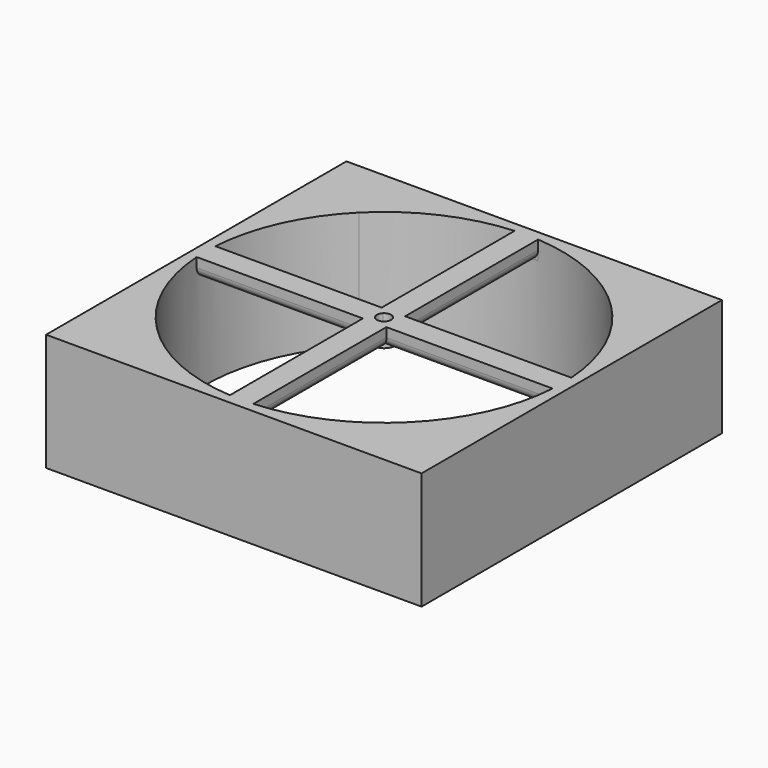
from build123d import *

# Parameters (mm, degrees)
F0_W          = 80
F0_H          = 80
F1_DEPTH      = 25
F3_DEPTH      = 25
F4_W          = 37.5
F4_H          = 5
F4_W_2        = 5
F4_H_2        = 37.5
F5_DEPTH      = 4
F6_T4_DEPTH   = 40.4176739793
F6_S5_R       = 38
F6_T6_DEPTH   = 22
F6_T10_DEPTH  = 40.4176739793
F6_S11_R      = 38
F6_T12_DEPTH  = 22
F6_T16_DEPTH  = 40.4176739793
F6_S17_R      = 38
F6_T18_DEPTH  = 22
F6_T22_DEPTH  = 40.4176739793
F6_S23_R      = 38
F6_T24_DEPTH  = 22
F6_T28_DEPTH  = 40.4176739793
F6_S29_R      = 38
F6_T30_DEPTH  = 22
F6_T34_DEPTH  = 40.4176739793
F6_S35_R      = 38
F6_T36_DEPTH  = 22
F6_T40_DEPTH  = 40.4176739793
F6_S41_R      = 38
F6_T42_DEPTH  = 22
F6_T46_DEPTH  = 40.4176739793
F6_S47_R      = 38
F6_T48_DEPTH  = 22
F6_T53_DEPTH  = 45.4176739793
F6_S54_R      = 1.5
F6_T55_DEPTH  = 24
F6_T59_DEPTH  = 45.4176739793
F6_S60_R      = 1.5
F6_T61_DEPTH  = 24
F6_T68_DEPTH  = 45.4176739793
F6_S69_R      = 1.5
F6_T70_DEPTH  = 24
F6_T74_DEPTH  = 45.4176739793
F6_S75_R      = 1.5
F6_T76_DEPTH  = 24
F6_T83_DEPTH  = 45.4176739793
F6_S85_R      = 1.5
F6_T86_DEPTH  = 24
F6_T89_DEPTH  = 45.4176739793
F6_S91_R      = 1.5
F6_T92_DEPTH  = 24
F6_T98_DEPTH  = 45.4176739793
F6_S99_R      = 1.5
F6_T100_DEPTH = 24
F6_T104_DEPTH = 45.4176739793
F6_S105_R     = 1.5
F6_T106_DEPTH = 24
F7_R          = 2.4952367962
F8_DEPTH      = 0.5


# Not quite as in the source:
# - a fillet or chamfer that OpenCascade refuses, or shapes differently, is made with other operations: its cross-section is extruded or revolved along the edge and cut away or added


with BuildPart() as f1:
    # F0 (on Top) → F1 (new body)
    with BuildSketch(Plane.XY):
        with Locations((-5.8039426804, 2.9257544003)):
            Rectangle(F0_W, F0_H)
    extrude(amount=F1_DEPTH)

    # F2 (on face) → F3 (cut)
    with BuildSketch(Plane.XY.offset(25)):
        with BuildLine():
            ThreePointArc((21.0661150047, 29.7958120854), (-5.8039426804, 40.9257544003), (-32.6740003654, 29.7958120854))
            Line((-32.6740003654, 29.7958120854), (-5.8039426804, 2.9257544003))
            Line((-5.8039426804, 2.9257544003), (21.0661150047, 29.7958120854))
        make_face()
        with BuildLine():
            Line((-5.8039426804, 2.9257544003), (-32.6740003654, 29.7958120854))
            ThreePointArc((-32.6740003654, 29.7958120854), (-43.8039426804, 2.9257544003), (-32.6740003654, -23.9443032848))
            Line((-32.6740003654, -23.9443032848), (-5.8039426804, 2.9257544003))
        make_face()
        with BuildLine():
            Line((21.0661150047, 29.7958120854), (-5.8039426804, 2.9257544003))
            Line((-5.8039426804, 2.9257544003), (21.0661150047, -23.9443032848))
            ThreePointArc((21.0661150047, -23.9443032848), (29.3034795551, -11.6162160296), (32.1960573196, 2.9257544003))
            ThreePointArc((32.1960573196, 2.9257544003), (29.3034795551, 17.4677248302), (21.0661150047, 29.7958120854))
        make_face()
        with BuildLine():
            Line((21.0661150047, -23.9443032848), (-5.8039426804, 2.9257544003))
            Line((-5.8039426804, 2.9257544003), (-32.6740003654, -23.9443032848))
            ThreePointArc((-32.6740003654, -23.9443032848), (-5.8039426804, -35.0742455997), (21.0661150047, -23.9443032848))
        make_face()
    extrude(amount=-F3_DEPTH, mode=Mode.SUBTRACT)

    # F4 (on face) → F5 (join)
    with BuildSketch(Plane.XY.offset(25)):
        Polygon((-8.3039426804, -37.0742455997), (-5.8039426804, -37.0742455997), (-3.3039426804, -37.0742455997), (-3.3039426804, 0.4257544003), (-8.3039426804, 0.4257544003), align=None)
        with Locations((-27.0539426804, 2.9257544003)):
            Rectangle(F4_W, F4_H)
        with BuildLine():
            Line((-6.8646028521, 1.8650942285), (-8.3039426804, 0.4257544003))
            Line((-8.3039426804, 0.4257544003), (-3.3039426804, 0.4257544003))
            Line((-3.3039426804, 0.4257544003), (-4.7432825086, 1.8650942285))
            ThreePointArc((-4.7432825086, 1.8650942285), (-5.8039426804, 1.4257544003), (-6.8646028521, 1.8650942285))
        make_face()
        with BuildLine():
            Line((-8.3039426804, 5.4257544003), (-8.3039426804, 0.4257544003))
            Line((-8.3039426804, 0.4257544003), (-6.8646028521, 1.8650942285))
            ThreePointArc((-6.8646028521, 1.8650942285), (-7.3039426804, 2.9257544003), (-6.8646028521, 3.9864145721))
            Line((-6.8646028521, 3.9864145721), (-8.3039426804, 5.4257544003))
        make_face()
        with BuildLine():
            Line((-4.7432825086, 1.8650942285), (-3.3039426804, 0.4257544003))
            Line((-3.3039426804, 0.4257544003), (-3.3039426804, 5.4257544003))
            Line((-3.3039426804, 5.4257544003), (-4.7432825086, 3.9864145721))
            ThreePointArc((-4.7432825086, 3.9864145721), (-4.4181233816, 3.4997795488), (-4.3039426804, 2.9257544003))
            ThreePointArc((-4.3039426804, 2.9257544003), (-4.4181233816, 2.3517292517), (-4.7432825086, 1.8650942285))
        make_face()
        with Locations((15.4460573196, 2.9257544003)):
            Rectangle(F4_W, F4_H)
        with Locations((-5.8039426804, 24.1757544003)):
            Rectangle(F4_W_2, F4_H_2)
        with BuildLine():
            Line((-3.3039426804, 5.4257544003), (-8.3039426804, 5.4257544003))
            Line((-8.3039426804, 5.4257544003), (-6.8646028521, 3.9864145721))
            ThreePointArc((-6.8646028521, 3.9864145721), (-5.8039426804, 4.4257544003), (-4.7432825086, 3.9864145721))
            Line((-4.7432825086, 3.9864145721), (-3.3039426804, 5.4257544003))
        make_face()
    extrude(amount=-F5_DEPTH)

    # F6: fillet of radius 2 on 8 edges, made by hand


with BuildPart() as f6_tool2:
    # F6_s3 → F6_t4 (new body)
    with BuildSketch(Plane.XZ.offset(-5.4257544003)):
        with BuildLine():
            ThreePointArc((-5.3039426804, 21), (-3.889729118, 21.5857864376), (-3.3039426804, 23))
            Line((-3.3039426804, 23), (-3.3039426804, 21))
            Line((-3.3039426804, 21), (-5.3039426804, 21))
        make_face()
    extrude(amount=-F6_T4_DEPTH)

    # F6_s5 → F6_t6 (intersect, symmetric)
    with BuildSketch(Plane.XY.offset(22)):
        with Locations((-5.8039426804, 2.9257544003)):
            Circle(F6_S5_R)
    extrude(amount=F6_T6_DEPTH, both=True, mode=Mode.INTERSECT)


with BuildPart() as f1_1:
    add(f1.part)

    # F6_t1: cut F6_tool2
    add(f6_tool2.part, mode=Mode.SUBTRACT)


with BuildPart() as f6_tool8:
    # F6_s9 → F6_t10 (new body)
    with BuildSketch(Plane.XZ.offset(-0.4257544003)):
        with BuildLine():
            ThreePointArc((-6.3039426804, 21), (-7.7181562427, 21.5857864376), (-8.3039426804, 23))
            Line((-8.3039426804, 23), (-8.3039426804, 21))
            Line((-8.3039426804, 21), (-6.3039426804, 21))
        make_face()
    extrude(amount=F6_T10_DEPTH)

    # F6_s11 → F6_t12 (intersect, symmetric)
    with BuildSketch(Plane.XY.offset(22)):
        with Locations((-5.8039426804, 2.9257544003)):
            Circle(F6_S11_R)
    extrude(amount=F6_T12_DEPTH, both=True, mode=Mode.INTERSECT)


with BuildPart() as f1_2:
    add(f1_1.part)

    # F6_t7: cut F6_tool8
    add(f6_tool8.part, mode=Mode.SUBTRACT)


with BuildPart() as f6_tool14:
    # F6_s15 → F6_t16 (new body)
    with BuildSketch(Plane.YZ.offset(-48.7216166597)):
        with BuildLine():
            ThreePointArc((2.4257544003, 21), (1.0115408379, 21.5857864376), (0.4257544003, 23))
            Line((0.4257544003, 23), (0.4257544003, 21))
            Line((0.4257544003, 21), (2.4257544003, 21))
        make_face()
    extrude(amount=F6_T16_DEPTH)

    # F6_s17 → F6_t18 (intersect, symmetric)
    with BuildSketch(Plane.XY.offset(22)):
        with Locations((-5.8039426804, 2.9257544003)):
            Circle(F6_S17_R)
    extrude(amount=F6_T18_DEPTH, both=True, mode=Mode.INTERSECT)


with BuildPart() as f1_3:
    add(f1_2.part)

    # F6_t13: cut F6_tool14
    add(f6_tool14.part, mode=Mode.SUBTRACT)


with BuildPart() as f6_tool20:
    # F6_s21 → F6_t22 (new body)
    with BuildSketch(Plane.YZ.offset(37.1137312989)):
        with BuildLine():
            ThreePointArc((3.4257544003, 21), (4.8399679627, 21.5857864376), (5.4257544003, 23))
            Line((5.4257544003, 23), (5.4257544003, 21))
            Line((5.4257544003, 21), (3.4257544003, 21))
        make_face()
    extrude(amount=-F6_T22_DEPTH)

    # F6_s23 → F6_t24 (intersect, symmetric)
    with BuildSketch(Plane.XY.offset(22)):
        with Locations((-5.8039426804, 2.9257544003)):
            Circle(F6_S23_R)
    extrude(amount=F6_T24_DEPTH, both=True, mode=Mode.INTERSECT)


with BuildPart() as f1_4:
    add(f1_3.part)

    # F6_t19: cut F6_tool20
    add(f6_tool20.part, mode=Mode.SUBTRACT)


with BuildPart() as f6_tool26:
    # F6_s27 → F6_t28 (new body)
    with BuildSketch(Plane.YZ.offset(-3.3039426804)):
        with BuildLine():
            ThreePointArc((2.4257544003, 21), (1.0115408379, 21.5857864376), (0.4257544003, 23))
            Line((0.4257544003, 23), (0.4257544003, 21))
            Line((0.4257544003, 21), (2.4257544003, 21))
        make_face()
    extrude(amount=F6_T28_DEPTH)

    # F6_s29 → F6_t30 (intersect, symmetric)
    with BuildSketch(Plane.XY.offset(22)):
        with Locations((-5.8039426804, 2.9257544003)):
            Circle(F6_S29_R)
    extrude(amount=F6_T30_DEPTH, both=True, mode=Mode.INTERSECT)


with BuildPart() as f1_5:
    add(f1_4.part)

    # F6_t25: cut F6_tool26
    add(f6_tool26.part, mode=Mode.SUBTRACT)


with BuildPart() as f6_tool32:
    # F6_s33 → F6_t34 (new body)
    with BuildSketch(Plane.YZ.offset(-8.3039426804)):
        with BuildLine():
            ThreePointArc((3.4257544003, 21), (4.8399679627, 21.5857864376), (5.4257544003, 23))
            Line((5.4257544003, 23), (5.4257544003, 21))
            Line((5.4257544003, 21), (3.4257544003, 21))
        make_face()
    extrude(amount=-F6_T34_DEPTH)

    # F6_s35 → F6_t36 (intersect, symmetric)
    with BuildSketch(Plane.XY.offset(22)):
        with Locations((-5.8039426804, 2.9257544003)):
            Circle(F6_S35_R)
    extrude(amount=F6_T36_DEPTH, both=True, mode=Mode.INTERSECT)


with BuildPart() as f1_6:
    add(f1_5.part)

    # F6_t31: cut F6_tool32
    add(f6_tool32.part, mode=Mode.SUBTRACT)


with BuildPart() as f6_tool38:
    # F6_s39 → F6_t40 (new body)
    with BuildSketch(Plane.XZ.offset(39.991919579)):
        with BuildLine():
            ThreePointArc((-3.3039426804, 23), (-3.889729118, 21.5857864376), (-5.3039426804, 21))
            Line((-5.3039426804, 21), (-3.3039426804, 21))
            Line((-3.3039426804, 21), (-3.3039426804, 23))
        make_face()
    extrude(amount=-F6_T40_DEPTH)

    # F6_s41 → F6_t42 (intersect, symmetric)
    with BuildSketch(Plane.XY.offset(22)):
        with Locations((-5.8039426804, 2.9257544003)):
            Circle(F6_S41_R)
    extrude(amount=F6_T42_DEPTH, both=True, mode=Mode.INTERSECT)


with BuildPart() as f1_7:
    add(f1_6.part)

    # F6_t37: cut F6_tool38
    add(f6_tool38.part, mode=Mode.SUBTRACT)


with BuildPart() as f6_tool44:
    # F6_s45 → F6_t46 (new body)
    with BuildSketch(Plane.XZ.offset(-45.8434283796)):
        with BuildLine():
            ThreePointArc((-6.3039426804, 21), (-7.7181562427, 21.5857864376), (-8.3039426804, 23))
            Line((-8.3039426804, 23), (-8.3039426804, 21))
            Line((-8.3039426804, 21), (-6.3039426804, 21))
        make_face()
    extrude(amount=F6_T46_DEPTH)

    # F6_s47 → F6_t48 (intersect, symmetric)
    with BuildSketch(Plane.XY.offset(22)):
        with Locations((-5.8039426804, 2.9257544003)):
            Circle(F6_S47_R)
    extrude(amount=F6_T48_DEPTH, both=True, mode=Mode.INTERSECT)


with BuildPart() as f1_8:
    add(f1_7.part)

    # F6_t43: cut F6_tool44
    add(f6_tool44.part, mode=Mode.SUBTRACT)


with BuildPart() as f6_tool51:
    # F6_s52 → F6_t53 (new body)
    with BuildSketch(Plane.XZ.offset(-0.4257544003)):
        with BuildLine():
            ThreePointArc((-5.3039426804, 21), (-3.889729118, 21.5857864376), (-3.3039426804, 23))
            Line((-3.3039426804, 23), (-3.3039426804, 21))
            Line((-3.3039426804, 21), (-5.3039426804, 21))
        make_face()
    extrude(amount=-F6_T53_DEPTH)

    # F6_s54 → F6_t55 (cut, symmetric)
    with BuildSketch(Plane.XY.offset(22)):
        with Locations((-5.8039426804, 2.9257544003)):
            Circle(F6_S54_R)
    extrude(amount=F6_T55_DEPTH, both=True, mode=Mode.SUBTRACT)

    split(bisect_by=Plane.XZ.offset(-5.4257544003), keep=Keep.TOP)


with BuildPart() as f6_tool57:
    # F6_s58 → F6_t59 (new body)
    with BuildSketch(Plane.YZ.offset(37.1137312989)):
        with BuildLine():
            ThreePointArc((3.4257544003, 21), (4.8399679627, 21.5857864376), (5.4257544003, 23))
            Line((5.4257544003, 23), (5.4257544003, 21))
            Line((5.4257544003, 21), (3.4257544003, 21))
        make_face()
    extrude(amount=-F6_T59_DEPTH)

    # F6_s60 → F6_t61 (cut, symmetric)
    with BuildSketch(Plane.XY.offset(22)):
        with Locations((-5.8039426804, 2.9257544003)):
            Circle(F6_S60_R)
    extrude(amount=F6_T61_DEPTH, both=True, mode=Mode.SUBTRACT)

    split(bisect_by=Plane.YZ.offset(-3.3039426804), keep=Keep.BOTTOM)


with BuildPart() as f6_tool51_1:
    add(f6_tool51.part)

    # F6_t63: intersect F6_tool57
    add(f6_tool57.part, mode=Mode.INTERSECT)


with BuildPart() as f1_9:
    add(f1_8.part)

    # F6_t49: cut F6_tool51
    add(f6_tool51_1.part, mode=Mode.SUBTRACT)


with BuildPart() as f6_tool66:
    # F6_s67 → F6_t68 (new body)
    with BuildSketch(Plane.YZ.offset(-48.7216166597)):
        with BuildLine():
            ThreePointArc((2.4257544003, 21), (1.0115408379, 21.5857864376), (0.4257544003, 23))
            Line((0.4257544003, 23), (0.4257544003, 21))
            Line((0.4257544003, 21), (2.4257544003, 21))
        make_face()
    extrude(amount=F6_T68_DEPTH)

    # F6_s69 → F6_t70 (cut, symmetric)
    with BuildSketch(Plane.XY.offset(22)):
        with Locations((-5.8039426804, 2.9257544003)):
            Circle(F6_S69_R)
    extrude(amount=F6_T70_DEPTH, both=True, mode=Mode.SUBTRACT)

    split(bisect_by=Plane.YZ.offset(-8.3039426804), keep=Keep.TOP)


with BuildPart() as f6_tool72:
    # F6_s73 → F6_t74 (new body)
    with BuildSketch(Plane.XZ.offset(-5.4257544003)):
        with BuildLine():
            ThreePointArc((-6.3039426804, 21), (-7.7181562427, 21.5857864376), (-8.3039426804, 23))
            Line((-8.3039426804, 23), (-8.3039426804, 21))
            Line((-8.3039426804, 21), (-6.3039426804, 21))
        make_face()
    extrude(amount=F6_T74_DEPTH)

    # F6_s75 → F6_t76 (cut, symmetric)
    with BuildSketch(Plane.XY.offset(22)):
        with Locations((-5.8039426804, 2.9257544003)):
            Circle(F6_S75_R)
    extrude(amount=F6_T76_DEPTH, both=True, mode=Mode.SUBTRACT)

    split(bisect_by=Plane.XZ.offset(-0.4257544003), keep=Keep.BOTTOM)


with BuildPart() as f6_tool66_1:
    add(f6_tool66.part)

    # F6_t78: intersect F6_tool72
    add(f6_tool72.part, mode=Mode.INTERSECT)


with BuildPart() as f1_10:
    add(f1_9.part)

    # F6_t64: cut F6_tool66
    add(f6_tool66_1.part, mode=Mode.SUBTRACT)


with BuildPart() as f6_tool81:
    # F6_s82 → F6_t83 (new body)
    with BuildSketch(Plane.XZ.offset(39.991919579)):
        with BuildLine():
            ThreePointArc((-3.3039426804, 23), (-3.889729118, 21.5857864376), (-5.3039426804, 21))
            Line((-5.3039426804, 21), (-3.3039426804, 21))
            Line((-3.3039426804, 21), (-3.3039426804, 23))
        make_face()
    extrude(amount=-F6_T83_DEPTH)

    split(bisect_by=Plane.XZ.offset(-0.4257544003), keep=Keep.BOTTOM)

    # F6_s85 → F6_t86 (cut, symmetric)
    with BuildSketch(Plane.XY.offset(22)):
        with Locations((-5.8039426804, 2.9257544003)):
            Circle(F6_S85_R)
    extrude(amount=F6_T86_DEPTH, both=True, mode=Mode.SUBTRACT)


with BuildPart() as f6_tool87:
    # F6_s88 → F6_t89 (new body)
    with BuildSketch(Plane.YZ.offset(-8.3039426804)):
        with BuildLine():
            ThreePointArc((2.4257544003, 21), (1.0115408379, 21.5857864376), (0.4257544003, 23))
            Line((0.4257544003, 23), (0.4257544003, 21))
            Line((0.4257544003, 21), (2.4257544003, 21))
        make_face()
    extrude(amount=F6_T89_DEPTH)

    split(bisect_by=Plane.YZ.offset(-3.3039426804), keep=Keep.BOTTOM)

    # F6_s91 → F6_t92 (cut, symmetric)
    with BuildSketch(Plane.XY.offset(22)):
        with Locations((-5.8039426804, 2.9257544003)):
            Circle(F6_S91_R)
    extrude(amount=F6_T92_DEPTH, both=True, mode=Mode.SUBTRACT)


with BuildPart() as f6_tool81_1:
    add(f6_tool81.part)

    # F6_t93: intersect F6_tool87
    add(f6_tool87.part, mode=Mode.INTERSECT)


with BuildPart() as f1_11:
    add(f1_10.part)

    # F6_t79: cut F6_tool81
    add(f6_tool81_1.part, mode=Mode.SUBTRACT)


with BuildPart() as f6_tool96:
    # F6_s97 → F6_t98 (new body)
    with BuildSketch(Plane.YZ.offset(-3.3039426804)):
        with BuildLine():
            ThreePointArc((3.4257544003, 21), (4.8399679627, 21.5857864376), (5.4257544003, 23))
            Line((5.4257544003, 23), (5.4257544003, 21))
            Line((5.4257544003, 21), (3.4257544003, 21))
        make_face()
    extrude(amount=-F6_T98_DEPTH)

    # F6_s99 → F6_t100 (cut, symmetric)
    with BuildSketch(Plane.XY.offset(22)):
        with Locations((-5.8039426804, 2.9257544003)):
            Circle(F6_S99_R)
    extrude(amount=F6_T100_DEPTH, both=True, mode=Mode.SUBTRACT)

    split(bisect_by=Plane.YZ.offset(-8.3039426804), keep=Keep.TOP)


with BuildPart() as f6_tool102:
    # F6_s103 → F6_t104 (new body)
    with BuildSketch(Plane.XZ.offset(-45.8434283796)):
        with BuildLine():
            ThreePointArc((-6.3039426804, 21), (-7.7181562427, 21.5857864376), (-8.3039426804, 23))
            Line((-8.3039426804, 23), (-8.3039426804, 21))
            Line((-8.3039426804, 21), (-6.3039426804, 21))
        make_face()
    extrude(amount=F6_T104_DEPTH)

    # F6_s105 → F6_t106 (cut, symmetric)
    with BuildSketch(Plane.XY.offset(22)):
        with Locations((-5.8039426804, 2.9257544003)):
            Circle(F6_S105_R)
    extrude(amount=F6_T106_DEPTH, both=True, mode=Mode.SUBTRACT)

    split(bisect_by=Plane.XZ.offset(-5.4257544003), keep=Keep.TOP)


with BuildPart() as f6_tool96_1:
    add(f6_tool96.part)

    # F6_t108: intersect F6_tool102
    add(f6_tool102.part, mode=Mode.INTERSECT)


with BuildPart() as f1_12:
    add(f1_11.part)

    # F6_t94: cut F6_tool96
    add(f6_tool96_1.part, mode=Mode.SUBTRACT)

    # F7 (on face) → F8 (join, symmetric)
    with BuildSketch(Plane(origin=(0, 0, 21), x_dir=(1, 0, 0), z_dir=(0, 0, -1))):
        with Locations((-5.8039426804, -2.9257544003)):
            Circle(F7_R)
        with BuildLine():
            ThreePointArc((-5.8039426804, -4.4257544003), (-6.8646028521, -1.8650942285), (-4.3039426804, -2.9257544003))
            ThreePointArc((-4.3039426804, -2.9257544003), (-4.7432825086, -3.9864145721), (-5.8039426804, -4.4257544003))
        make_face(mode=Mode.SUBTRACT)
    extrude(amount=F8_DEPTH, both=True)


solid = f1_12.part
